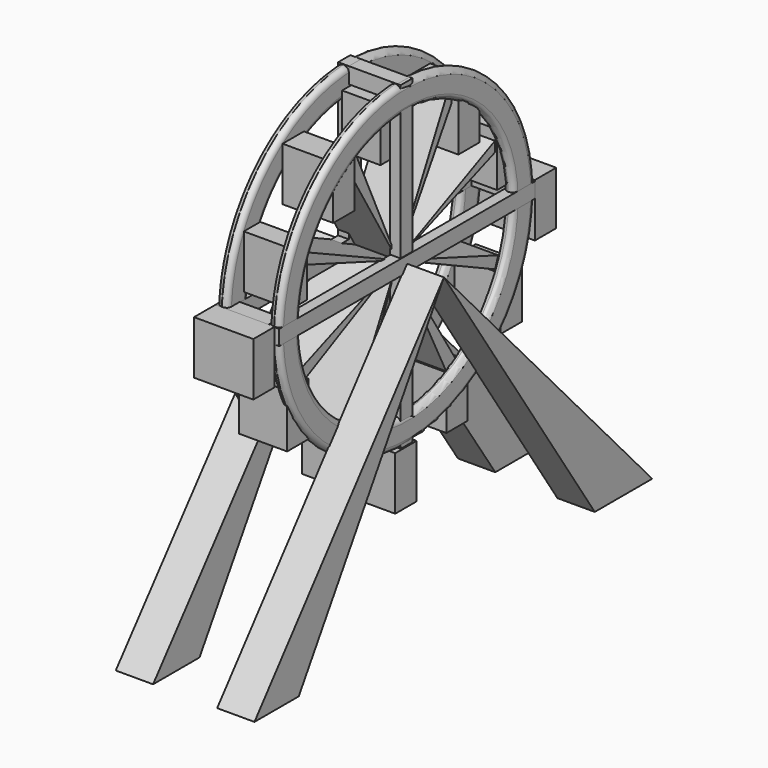
from build123d import *

# Parameters (mm, degrees)
F0_R      = 76.2
F1_DEPTH  = 5.08
F2_R      = 63.5
F3_DEPTH  = 28.448
F8_R      = 2.54
F9_R      = 2.53999
F10_R     = 2.54
F11_R     = 2.53999
F12_R     = 2.53999
F13_W     = 7.2420393117
F13_H     = 152.5342464447
F14_DEPTH = 5.08
F18_W     = 7.2420393117
F18_H     = 7.62
F19_DEPTH = 23.114
F20_W     = 7.2420393117
F20_H     = 7.62
F21_DEPTH = 21.59
F22_W     = 152.4
F22_H     = 7.242048
F23_DEPTH = 5.08
F25_W     = 7.5083374977
F25_H     = 7.5877550989
F26_DEPTH = 25.4
F27_W     = 6.6496804357
F27_H     = 7.1474232245
F28_DEPTH = 25.4
F29_W     = 28.258436572
F29_H     = 25.4
F30_DEPTH = 12.7
F31_W     = 30.48
F31_H     = 25.4
F32_DEPTH = 12.7
F33_W     = 30.3243320611
F33_H     = 12.7
F34_DEPTH = 25.4
F35_W     = 18.2815846842
F35_H     = 12.7
F36_DEPTH = 25.4
F38_DEPTH = 17.78
F40_DEPTH = 17.78
F42_DEPTH = 25.4
F43_W     = 12.7
F43_H     = 25.4
F44_DEPTH = 24.13
F45_W     = 9.7887781068
F45_H     = 25.4
F46_DEPTH = 22.352
F47_W     = 12.7
F47_H     = 25.4
F48_DEPTH = 22.86
F49_W     = 11.4898889749
F49_H     = 25.4
F50_DEPTH = 16.764
F51_W     = 12.7
F51_H     = 25.4
F52_DEPTH = 20.066
F53_W     = 12.7
F53_H     = 25.4
F54_DEPTH = 21.971
F55_W     = 12.7
F55_H     = 25.4
F56_DEPTH = 23.622
F57_W     = 11.43
F57_H     = 25.4
F58_DEPTH = 21.336


# Not quite as in the source:
# - a fillet or chamfer is up to 0.001 mm smaller than in the source, because OpenCascade refuses the exact size


with BuildPart() as f1:
    # F0 (on Right) → F1 (new body)
    with BuildSketch(Plane.YZ):
        Circle(F0_R)
    extrude(amount=F1_DEPTH)

    # F2 (on face) → F3 (cut, symmetric)
    with BuildSketch(Plane.YZ.offset(5.08)):
        Circle(F2_R)
    extrude(amount=F3_DEPTH, both=True, mode=Mode.SUBTRACT)


with BuildPart() as f5_1:
    # F5: copy of F1
    add(f1.part.moved(Location((9.398, 0, 0))))


with BuildPart() as f6_1:
    # F6: copy of F5_1
    add(f5_1.part.moved(Location((15.494, 0, 0))))

    # F12 (radius 2.54 in the source; OpenCascade refuses exactly that, so slightly less here)
    f12_edges = [f6_1.edges().sort_by_distance(p)[0] for p in [
        (24.892, -76.2, 0),
        (24.892, -63.5, 0),
        (29.972, -63.5, 0),
        (29.972, -76.2, 0),
    ]]
    fillet(f12_edges, radius=F12_R)


with BuildPart() as f1_1:
    add(f1.part)

    # F8
    f8_edges = [f1_1.edges().sort_by_distance(p)[0] for p in [
        (0, -76.2, 0),
    ]]
    fillet(f8_edges, radius=F8_R)

    # F9 (radius 2.54 in the source; OpenCascade refuses exactly that, so slightly less here)
    f9_edges = [f1_1.edges().sort_by_distance(p)[0] for p in [
        (5.08, -76.2, 0),
    ]]
    fillet(f9_edges, radius=F9_R)

    # F10
    f10_edges = [f1_1.edges().sort_by_distance(p)[0] for p in [
        (0, -63.5, 0),
    ]]
    fillet(f10_edges, radius=F10_R)

    # F11 (radius 2.54 in the source; OpenCascade refuses exactly that, so slightly less here)
    f11_edges = [f1_1.edges().sort_by_distance(p)[0] for p in [
        (5.08, -63.5, 0),
    ]]
    fillet(f11_edges, radius=F11_R)


with BuildPart() as f14:
    # F13 (on Right) → F14 (new body)
    with BuildSketch(Plane.YZ):
        Rectangle(F13_W, F13_H)
    extrude(amount=F14_DEPTH)


with BuildPart() as f15_1:
    # F15: copy of F14
    add(f14.part.moved(Location((17.018, 0, 0))))


with BuildPart() as f16_1:
    # F16: copy of F15_1
    add(f15_1.part.moved(Location((7.62, 0, 0))))


with BuildPart() as f19:
    # F18 (on face) → F19 (new body)
    with BuildSketch(Plane.YZ.offset(5.08)):
        with Locations((0, 72.4571232224)):
            Rectangle(F18_W, F18_H)
    extrude(amount=F19_DEPTH)

    # F35 (on face) → F36 (join)
    with BuildSketch(Plane(origin=(0, 0, 68.6471232224), x_dir=(1, 0, 0), z_dir=(0, 0, -1))):
        with Locations((15.3832314143, 2.7289803442)):
            Rectangle(F35_W, F35_H)
    extrude(amount=F36_DEPTH)


with BuildPart() as f21:
    # F20 (on face) → F21 (new body)
    with BuildSketch(Plane.YZ.offset(5.08)):
        with Locations((0, -72.4571232224)):
            Rectangle(F20_W, F20_H)
    extrude(amount=F21_DEPTH)


with BuildPart() as f23:
    # F22 (on Right) → F23 (new body)
    with BuildSketch(Plane.YZ):
        Rectangle(F22_W, F22_H)
    extrude(amount=F23_DEPTH)


with BuildPart() as f24_1:
    # F24: copy of F23
    add(f23.part.moved(Location((24.892, 0, 0))))


with BuildPart() as f26:
    # F25 (on face) → F26 (new body)
    with BuildSketch(Plane(origin=(24.892, 0, 0), x_dir=(0, -1, 0), z_dir=(-1, 0, 0))):
        with Locations((72.3730251193, 0.0060452148)):
            Rectangle(F25_W, F25_H)
    extrude(amount=F26_DEPTH)


with BuildPart() as f28:
    # F27 (on face) → F28 (new body)
    with BuildSketch(Plane(origin=(24.892, 0, 0), x_dir=(0, -1, 0), z_dir=(-1, 0, 0))):
        with Locations((-72.7413855493, -0.0455594854)):
            Rectangle(F27_W, F27_H)
    extrude(amount=F28_DEPTH)


with BuildPart() as f30:
    # F29 (on face) → F30 (new body)
    with BuildSketch(Plane.XZ.offset(76.1271938682)):
        with Locations((13.621218286, -8.9000772357)):
            Rectangle(F29_W, F29_H)
    extrude(amount=F30_DEPTH)


with BuildPart() as f32:
    # F31 (on face) → F32 (new body)
    with BuildSketch(Plane(origin=(0, 76.0662257671, 0), x_dir=(-1, 0, 0), z_dir=(0, 1, 0))):
        with Locations((-14.732, -8.4941469923)):
            Rectangle(F31_W, F31_H)
    extrude(amount=F32_DEPTH)


with BuildPart() as f34:
    # F33 (on face) → F34 (new body)
    with BuildSketch(Plane(origin=(0, 0, -76.2671232224), x_dir=(1, 0, 0), z_dir=(0, 0, -1))):
        with Locations((15.1621660306, 1.1962651973)):
            Rectangle(F33_W, F33_H)
    extrude(amount=F34_DEPTH)


with BuildPart() as f38:
    # F37 (on face) → F38 (new body)
    with BuildSketch(Plane.YZ.offset(29.718)):
        Polygon((-86.4798873663, -140.5976116657), (0, 0), (-112.8344163299, -140.5976116657), align=None)
    extrude(amount=F38_DEPTH)


with BuildPart() as f38b:
    # F37 (on face) → F38, piece 2 (new body)
    with BuildSketch(Plane.YZ.offset(29.718)):
        Polygon((124.0512356162, -134.9076479673), (0, 0), (89.8195281625, -134.9076479673), align=None)
    extrude(amount=F38_DEPTH)


with BuildPart() as f40:
    # F39 (on face) → F40 (new body)
    with BuildSketch(Plane.YZ):
        Polygon((122.7524504066, -133.7626874447), (0, 0), (89.9559929967, -133.7626874447), align=None)
    extrude(amount=-F40_DEPTH)


with BuildPart() as f40b:
    # F39 (on face) → F40, piece 2 (new body)
    with BuildSketch(Plane.YZ):
        Polygon((-86.2078368664, -139.8534625769), (0, 0), (-113.850556314, -139.8534625769), align=None)
    extrude(amount=-F40_DEPTH)


with BuildPart() as f42:
    # F41 (on Right) → F42 (new body)
    with BuildSketch(Plane.YZ):
        Polygon((28.9433617145, 56.614741683), (0, 0), (33.1683402025, 54.4547904586), align=None)
    extrude(amount=F42_DEPTH)


with BuildPart() as f42b:
    # F41 (on Right) → F42, piece 2 (new body)
    with BuildSketch(Plane.YZ):
        Polygon((58.0660738051, 26.5383217484), (0, 0), (59.969408968, 22.373808216), align=None)
    extrude(amount=F42_DEPTH)


with BuildPart() as f42c:
    # F41 (on Right) → F42, piece 3 (new body)
    with BuildSketch(Plane.YZ):
        Polygon((-31.9048750725, 53.8588724908), (0, 0), (-25.8750098298, 56.614741683), align=None)
    extrude(amount=F42_DEPTH)


with BuildPart() as f42d:
    # F41 (on Right) → F42, piece 4 (new body)
    with BuildSketch(Plane.YZ):
        Polygon((-58.9155611091, 21.908053265), (0, 0), (-56.7502938211, 26.5383217484), align=None)
    extrude(amount=F42_DEPTH)


with BuildPart() as f42e:
    # F41 (on Right) → F42, piece 5 (new body)
    with BuildSketch(Plane.YZ):
        Polygon((-56.437973012, -28.0128466662), (0, 0), (-58.9155611091, -22.5918628275), align=None)
    extrude(amount=F42_DEPTH)


with BuildPart() as f42f:
    # F41 (on Right) → F42, piece 6 (new body)
    with BuildSketch(Plane.YZ):
        Polygon((-25.578148865, -59.0636329811), (0, 0), (-29.4577805545, -57.6209720592), align=None)
    extrude(amount=F42_DEPTH)


with BuildPart() as f42g:
    # F41 (on Right) → F42, piece 7 (new body)
    with BuildSketch(Plane.YZ):
        Polygon((34.3674241515, -55.0995962899), (0, 0), (28.9433617145, -58.3126979839), align=None)
    extrude(amount=F42_DEPTH)


with BuildPart() as f42h:
    # F41 (on Right) → F42, piece 8 (new body)
    with BuildSketch(Plane.YZ):
        Polygon((59.969408968, -22.299931991), (0, 0), (58.0660738051, -27.4184177709), align=None)
    extrude(amount=F42_DEPTH)


with BuildPart() as f44:
    # F43 (on face) → F44 (new body)
    with BuildSketch(Plane.YZ.offset(5.08)):
        with Locations((-36.7189122477, 47.0567100651)):
            Rectangle(F43_W, F43_H)
    extrude(amount=F44_DEPTH)


with BuildPart() as f46:
    # F45 (on face) → F46 (new body)
    with BuildSketch(Plane.YZ.offset(5.08)):
        with Locations((-61.2684678192, 19.6770284376)):
            Rectangle(F45_W, F45_H)
    extrude(amount=F46_DEPTH)


with BuildPart() as f48:
    # F47 (on face) → F48 (new body)
    with BuildSketch(Plane.YZ.offset(5.08)):
        with Locations((-62.57914298, -38.6724632649)):
            Rectangle(F47_W, F47_H)
    extrude(amount=F48_DEPTH)


with BuildPart() as f50:
    # F49 (on face) → F50 (new body)
    with BuildSketch(Plane.YZ.offset(5.08)):
        with Locations((-25.7132970617, -70.7660024337)):
            Rectangle(F49_W, F49_H)
    extrude(amount=F50_DEPTH)


with BuildPart() as f52:
    # F51 (on face) → F52 (new body)
    with BuildSketch(Plane.YZ.offset(5.08)):
        with Locations((35.7584207724, -71.830587581)):
            Rectangle(F51_W, F51_H)
    extrude(amount=F52_DEPTH)


with BuildPart() as f54:
    # F53 (on face) → F54 (new body)
    with BuildSketch(Plane.YZ.offset(5.08)):
        with Locations((65.6234703966, -41.8193630964)):
            Rectangle(F53_W, F53_H)
    extrude(amount=F54_DEPTH)


with BuildPart() as f56:
    # F55 (on face) → F56 (new body)
    with BuildSketch(Plane.YZ.offset(5.08)):
        with Locations((38.4269728878, 45.0265052671)):
            Rectangle(F55_W, F55_H)
    extrude(amount=F56_DEPTH)


with BuildPart() as f58:
    # F57 (on face) → F58 (new body)
    with BuildSketch(Plane.YZ.offset(5.08)):
        with Locations((63.7174061525, 18.8753460872)):
            Rectangle(F57_W, F57_H)
    extrude(amount=F58_DEPTH)


solid = Compound([f6_1.part, f1_1.part, f14.part, f16_1.part, f19.part, f21.part, f23.part, f24_1.part, f26.part, f28.part, f30.part, f32.part, f34.part, f38.part, f38b.part, f40.part, f40b.part, f42.part, f42b.part, f42c.part, f42d.part, f42e.part, f42f.part, f42g.part, f42h.part, f44.part, f46.part, f48.part, f50.part, f52.part, f54.part, f56.part, f58.part])
